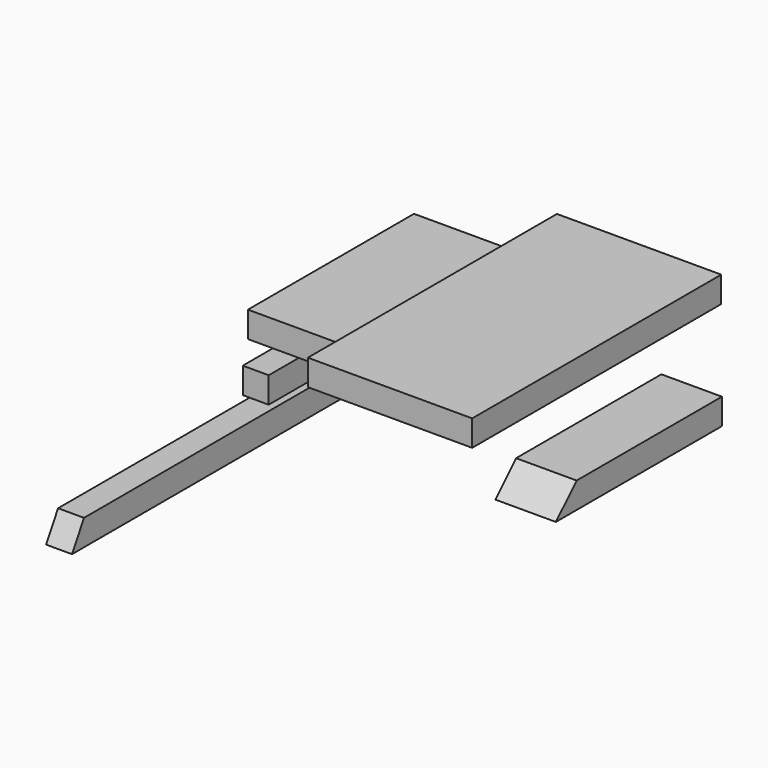
from build123d import *

# Parameters (mm, degrees)
F0_W         = 88.9
F0_H         = 38.1
F1_DEPTH     = 304.8
F3_W         = 139.7
F3_H         = 38.1
F4_DEPTH     = 304.8
F6_W         = 241.3
F6_H         = 38.1
F7_DEPTH     = 457.2
F8_W         = 38.1
F8_H         = 38.1
F9_DEPTH     = 304.8
F10_W        = 88.9
F10_H        = 38.1
F11_DEPTH    = 304.8
F12_SIZE     = 38.09999
F13_W        = 38.1
F13_H        = 38.1
F14_DEPTH    = 609.6
F15_T1_DEPTH = 265.7329697057


# Not quite as in the source:
# - a fillet or chamfer that OpenCascade refuses, or shapes differently, is made with other operations: its cross-section is extruded or revolved along the edge and cut away or added
# - a fillet or chamfer is up to 0.001 mm smaller than in the source, because OpenCascade refuses the exact size


with BuildPart() as f1:
    # F0 (on Front) → F1 (new body)
    with BuildSketch(Plane.XZ):
        with Locations((44.45, 19.05)):
            Rectangle(F0_W, F0_H)
    extrude(amount=F1_DEPTH)


with BuildPart() as f2_1:
    # F2: copy of F1
    add(f1.part.moved(Location((127, 0, 0))))


with BuildPart() as f4:
    # F3 (on Front) → F4 (new body)
    with BuildSketch(Plane.XZ):
        with Locations((-134.2311747432, 23.224890928)):
            Rectangle(F3_W, F3_H)
    extrude(amount=F4_DEPTH)


with BuildPart() as f7:
    # F6 (on Front) → F7 (new body)
    with BuildSketch(Plane.XZ):
        with Locations((126.5473598003, 91.3414934158)):
            Rectangle(F6_W, F6_H)
    extrude(amount=F7_DEPTH)


with BuildPart() as f9:
    # F8 (on Front) → F9 (new body)
    with BuildSketch(Plane.XZ):
        with Locations((-192.5818750143, -51.6675061107)):
            Rectangle(F8_W, F8_H)
    extrude(amount=F9_DEPTH)


with BuildPart() as f11:
    # F10 (on Front) → F11 (new body)
    with BuildSketch(Plane.XZ):
        with Locations((203.7315069914, -66.1231598377)):
            Rectangle(F10_W, F10_H)
    extrude(amount=F11_DEPTH)

    # F12 (size 38.1 in the source; OpenCascade refuses exactly that, so slightly less here)
    f12_edges = [f11.edges().sort_by_distance(p)[0] for p in [
        (203.731507, -304.8, -47.07316),
    ]]
    chamfer(f12_edges, length=F12_SIZE)


with BuildPart() as f14:
    # F13 (on Front) → F14 (new body)
    with BuildSketch(Plane.XZ):
        with Locations((-240.3054216385, -137.9403641939)):
            Rectangle(F13_W, F13_H)
    extrude(amount=F14_DEPTH)

    # F15: chamfer of 25.4 x 43.9940905122 on 1 edges, made by hand

    # F15_s2 → F15_t1 (cut)
    with BuildSketch(Plane.YZ.offset(-373.1719064913)):
        Polygon((-584.2, -118.8903641939), (-609.6, -162.8844547062), (-609.6, -118.8903641939), align=None)
    extrude(amount=F15_T1_DEPTH, mode=Mode.SUBTRACT)


solid = Compound([f1.part, f4.part, f7.part, f9.part, f11.part, f14.part])
